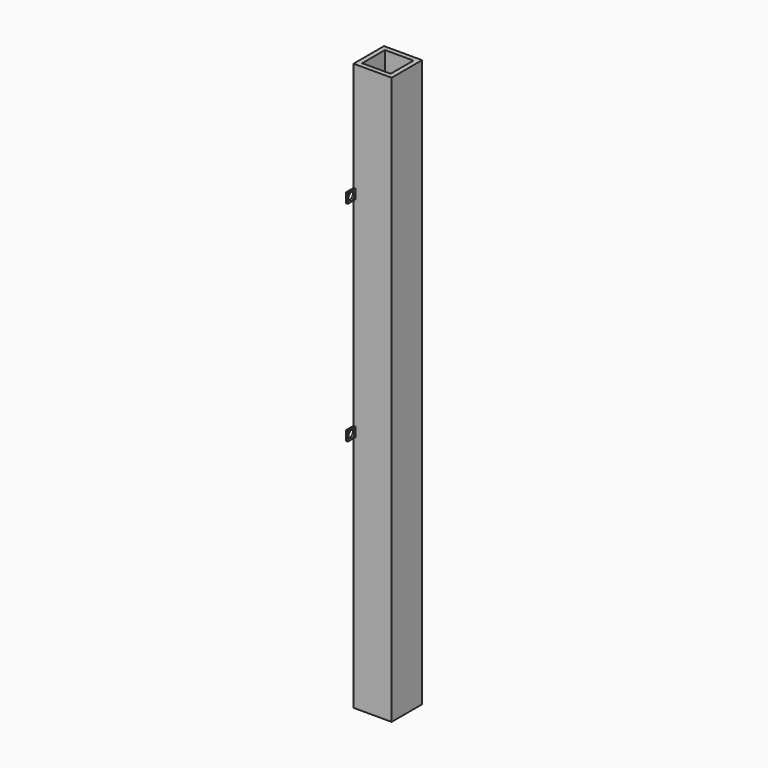
from build123d import *

# Parameters (mm, degrees)
F0_W     = 20
F0_H     = 298
F1_DEPTH = 20
F2_T     = -2.5
F3_W     = 5
F3_H     = 5
F4_DEPTH = 1
F5_D     = 4


# Not quite as in the source:
# - a feature names something its author has since deleted; it is built from what else it names


with BuildPart() as f1:
    # F0 (on Right) → F1 (new body)
    with BuildSketch(Plane.YZ):
        Rectangle(F0_W, F0_H)
    extrude(amount=F1_DEPTH)

    # F2
    f2_openings = [f1.faces().sort_by_distance(p)[0] for p in [
        (10, 0, 149),
    ]]
    offset(amount=F2_T, openings=f2_openings)

    # F3 (on face) → F4 (join)
    with BuildSketch(Plane(origin=(0, 0, 0), x_dir=(0, -1, 0), z_dir=(-1, 0, 0))):
        with Locations((12.5, 89)):
            Rectangle(F3_W, F3_H)
        with Locations((-12.5, 89)):
            Rectangle(F3_W, F3_H)
        with Locations((-12.5, -21)):
            Rectangle(F3_W, F3_H)
        with Locations((12.5, -21)):
            Rectangle(F3_W, F3_H)
    extrude(amount=-F4_DEPTH)

    # F5 (through all)
    with Locations(Plane(origin=(0, 0, 0), x_dir=(0, -1, 0), z_dir=(-1, 0, 0))):
        with Locations((-12.5, 89), (12.5, 89), (-12.5, -21), (12.5, -21)):
            Hole(F5_D / 2)


solid = f1.part
